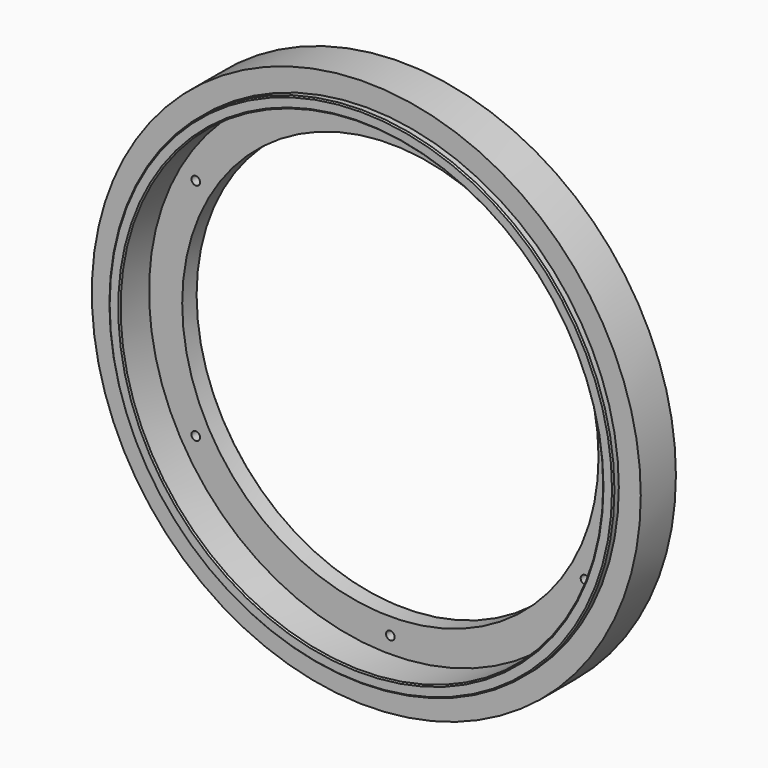
from build123d import *

# Parameters (mm, degrees)
F0_R             = 152.4
F0_R_2           = 120.396
F1_DEPTH         = 11.176
F2_R             = 152.4
F2_R_2           = 139.573
F3_DEPTH         = 21.336
F6_SIZE          = 0.762
F7_W             = 12.7
F7_H             = 25.4
F9_R             = 6.35
F10_DEPTH        = 4.7752
F10_COPIES_COUNT = 6
F11_R            = 2.4892
F12_DEPTH        = 25.4
F12_COPIES_COUNT = 6


# Not quite as in the source:
# - a pattern or mirror of a feature is missing from the dataset's text; its kind, count and spacing are read off the source's solid


with BuildPart() as f1:
    # F0 (on Front) → F1 (new body)
    with BuildSketch(Plane.XZ):
        Circle(F0_R)
        Circle(F0_R_2, mode=Mode.SUBTRACT)
    extrude(amount=-F1_DEPTH)

    # F2 (on face) → F3 (join)
    with BuildSketch(Plane.XZ):
        Circle(F2_R)
        Circle(F2_R_2, mode=Mode.SUBTRACT)
    extrude(amount=F3_DEPTH)

    # F4 (on Top) → F5 (revolve, cut)
    with BuildSketch(Plane.XY):
        Polygon((176.0028898716, -18.161), (176.0028898716, 8.001), (146.05, 8.001), (146.05, -18.161), (146.05, -21.336), (152.4, -21.336), (176.0028898716, -21.336), align=None)
    revolve(axis=Axis((0, -10.1678725332, 0), (0, -1, 0)), mode=Mode.SUBTRACT)

    # F6
    f6_edges = [f1.edges().sort_by_distance(p)[0] for p in [
        (-120.396, 11.176, 0),
        (-152.4, 11.176, 0),
        (-139.573, -21.336, 0),
        (-146.05, -21.336, 0),
        (146.05, -6.6675, 0),
    ]]
    chamfer(f6_edges, length=F6_SIZE)

    # F9 (on face) → F10 (cut)
    with BuildSketch(Plane(origin=(0, 11.176, 0), x_dir=(-1, 0, 0), z_dir=(0, 1, 0))):
        with Locations((0, 129.9845)):
            Circle(F9_R)
    f10 = extrude(amount=-F10_DEPTH, mode=Mode.SUBTRACT)

    # F10_copies: F10 ×6 about axis
    f10_copies_axis = Axis((0, 0, 0), (0, 1, 0))
    for i in range(1, F10_COPIES_COUNT):
        add(f10.rotate(f10_copies_axis, i * 360 / F10_COPIES_COUNT), mode=Mode.SUBTRACT)

    # F11 (on face) → F12 (cut)
    with BuildSketch(Plane(origin=(0, 11.176, 0), x_dir=(-1, 0, 0), z_dir=(0, 1, 0))):
        with Locations((0, 129.9845)):
            Circle(F11_R)
    f12 = extrude(amount=-F12_DEPTH, mode=Mode.SUBTRACT)

    # F12_copies: F12 ×6 about axis
    f12_copies_axis = Axis((0, 0, 0), (0, 1, 0))
    for i in range(1, F12_COPIES_COUNT):
        add(f12.rotate(f12_copies_axis, i * 360 / F12_COPIES_COUNT), mode=Mode.SUBTRACT)


with BuildPart() as f8:
    # F7 (on Top) → F8 (revolve)
    with BuildSketch(Plane.XY):
        with Locations((152.4, -4.699)):
            Rectangle(F7_W, F7_H)
    revolve(axis=Axis((0, -13.9294480905, 0), (0, -1, 0)))


solid = Compound([f1.part, f8.part])
